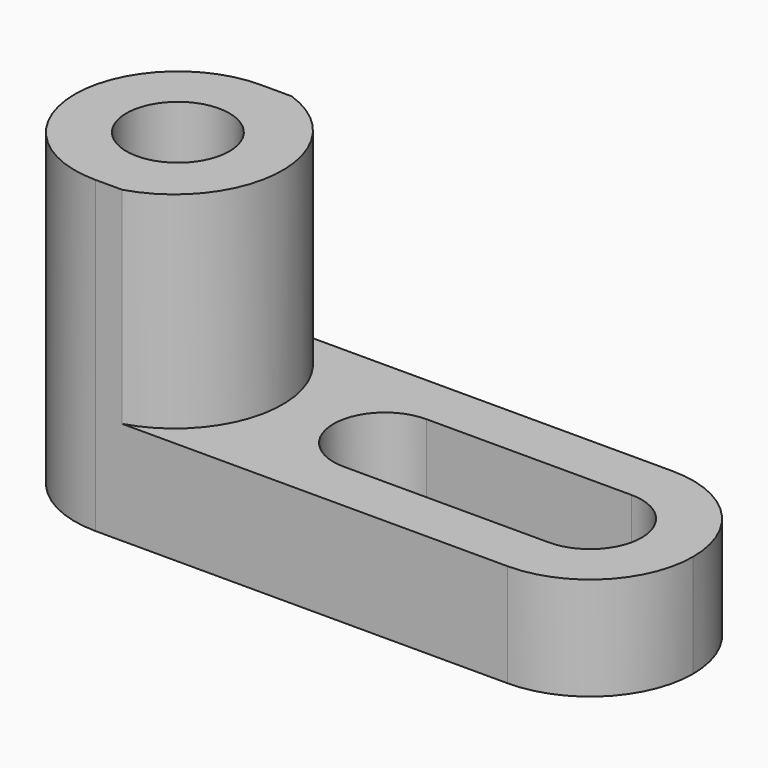
from build123d import *

# Parameters (mm, degrees)
F1_DEPTH = 25.4
F3_DEPTH = 25.4
F4_R     = 6.35
F5_DEPTH = 127
F7_DEPTH = 25.4
F9_DEPTH = 25.4


# Not quite as in the source:
# - a feature names something its author has since deleted; it is built from what else it names


with BuildPart() as f1:
    # F0 (on Front) → F1 (new body)
    with BuildSketch(Plane.XZ):
        Polygon((-28.758216656, 38.1), (-54.158216656, 38.1), (-54.158216656, 0), (22.041783344, 0), (22.041783344, 12.7), (-28.758216656, 12.7), align=None)
    extrude(amount=F1_DEPTH)

    # F2 (on face) → F3 (join)
    with BuildSketch(Plane.XY.offset(12.7)):
        with BuildLine():
            Line((-28.758216656, 0), (-28.758216656, -25.4))
            ThreePointArc((-28.758216656, -25.4), (-23.817550475, -12.7), (-28.758216656, 0))
        make_face()
    extrude(amount=F3_DEPTH)

    # F4 (on face) → F5 (cut)
    with BuildSketch(Plane.XY.offset(38.1)):
        with BuildLine():
            ThreePointArc((-54.158216656, -12.7), (-50.438472777, -3.7197438789), (-41.458216656, 0))
            Line((-41.458216656, 0), (-54.158216656, 0))
            Line((-54.158216656, 0), (-54.158216656, -12.7))
        make_face()
        with BuildLine():
            Line((-54.158216656, -25.4), (-41.458216656, -25.4))
            ThreePointArc((-41.458216656, -25.4), (-50.438472777, -21.6802561211), (-54.158216656, -12.7))
            Line((-54.158216656, -12.7), (-54.158216656, -25.4))
        make_face()
        with Locations((-41.458216656, -12.7)):
            Circle(F4_R)
    extrude(amount=-F5_DEPTH, mode=Mode.SUBTRACT)

    # F6 (on face) → F7 (cut)
    with BuildSketch(Plane.XY.offset(38.1)):
        with BuildLine():
            ThreePointArc((-37.5933498144, 0), (-28.6296169388, -12.9065923281), (-38.1607972085, -25.4))
            Line((-38.1607972085, -25.4), (-28.758216656, -25.4))
            ThreePointArc((-28.758216656, -25.4), (-23.817550475, -12.7), (-28.758216656, 0))
            Line((-28.758216656, 0), (-37.5933498144, 0))
        make_face()
    extrude(amount=-F7_DEPTH, mode=Mode.SUBTRACT)

    # F8 (on face) → F9 (cut)
    with BuildSketch(Plane.XY.offset(12.7)):
        with BuildLine():
            ThreePointArc((15.691783344, -12.7), (13.8319114046, -8.2098719395), (9.341783344, -6.35))
            ThreePointArc((9.341783344, -6.35), (2.991783344, -12.7), (9.341783344, -19.05))
            ThreePointArc((9.341783344, -19.05), (13.8319114046, -17.1901280605), (15.691783344, -12.7))
        make_face()
        with BuildLine():
            ThreePointArc((-15.9312973803, -6.35), (-11.4411693197, -8.2098719395), (-9.5812973803, -12.7))
            ThreePointArc((-9.5812973803, -12.7), (-11.4411693197, -17.1901280605), (-15.9312973803, -19.05))
            Line((-15.9312973803, -19.05), (9.341783344, -19.05))
            ThreePointArc((9.341783344, -19.05), (2.991783344, -12.7), (9.341783344, -6.35))
            Line((9.341783344, -6.35), (-15.9312973803, -6.35))
        make_face()
        with BuildLine():
            ThreePointArc((-15.9312973803, -19.05), (-11.4411693197, -17.1901280605), (-9.5812973803, -12.7))
            ThreePointArc((-9.5812973803, -12.7), (-11.4411693197, -8.2098719395), (-15.9312973803, -6.35))
            ThreePointArc((-15.9312973803, -6.35), (-22.2812973803, -12.7), (-15.9312973803, -19.05))
        make_face()
        with BuildLine():
            ThreePointArc((9.341783344, 0), (18.3220394651, -3.7197438789), (22.041783344, -12.7))
            Line((22.041783344, -12.7), (22.041783344, 0))
            Line((22.041783344, 0), (9.341783344, 0))
        make_face()
        with BuildLine():
            ThreePointArc((22.041783344, -12.7), (18.3220394651, -21.6802561211), (9.341783344, -25.4))
            Line((9.341783344, -25.4), (22.041783344, -25.4))
            Line((22.041783344, -25.4), (22.041783344, -12.7))
        make_face()
    extrude(amount=-F9_DEPTH, mode=Mode.SUBTRACT)


solid = f1.part
